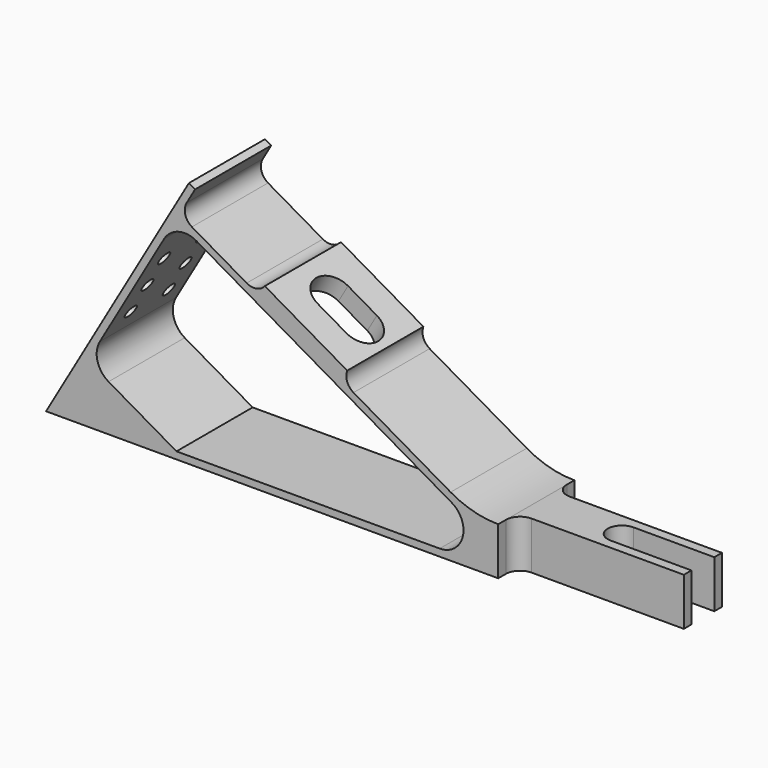
from build123d import *

# Parameters (mm, degrees)
F1_DEPTH    = 10
F2_T1_DEPTH = 20
F4_DEPTH    = 20.001
F5_W        = 35
F5_H        = 5
F6_DEPTH    = 10.001
F7_R        = 3
F9_DEPTH    = 10.001
F11_DEPTH   = 4
F12_R       = 5.5
F13_DEPTH   = 2
F14_R       = 4.25
F15_DEPTH   = 112.584302492
F16_R       = 1.395
F17_DEPTH   = 25


# Not quite as in the source:
# - a fillet or chamfer that OpenCascade refuses, or shapes differently, is made with other operations: its cross-section is extruded or revolved along the edge and cut away or added


with BuildPart() as f1:
    # F0 (on Front) → F1 (new body, symmetric)
    with BuildSketch(Plane.XZ):
        with BuildLine():
            Line((30, 51.9615242271), (0, 0))
            Line((0, 0), (130, 0))
            Line((130, 0), (130, 10))
            Line((130, 10), (95, 10))
            ThreePointArc((95, 10), (89.8236190979, 10.6814834742), (85, 12.6794919243))
            Line((85, 12.6794919243), (62.0314784198, 25.9403740415))
            Line((62.0314784198, 25.9403740415), (63.2814784198, 28.105437551))
            Line((63.2814784198, 28.105437551), (45.9609703441, 38.105437551))
            Line((45.9609703441, 38.105437551), (44.7109703441, 35.9403740415))
            Line((44.7109703441, 35.9403740415), (28.0394191624, 45.5656986041))
            Line((28.0394191624, 45.5656986041), (31.2990381057, 51.2115242271))
            Line((31.2990381057, 51.2115242271), (30, 51.9615242271))
        make_face()
    extrude(amount=F1_DEPTH, both=True)

    # F2: fillet of radius 3 on 3 edges, made by hand

    # F2_s2 → F2_t1 (join)
    with BuildSketch(Plane.XZ.offset(-10)):
        with BuildLine():
            ThreePointArc((63.2814784198, 28.105437551), (63.2705212044, 26.0433626604), (64.5932161113, 24.4613540958))
            Line((64.5932161113, 24.4613540958), (62.0314784198, 25.9403740415))
            Line((62.0314784198, 25.9403740415), (63.2814784198, 28.105437551))
        make_face()
        with BuildLine():
            ThreePointArc((42.1492326526, 37.4193939873), (44.180639712, 37.0649108788), (45.9609703441, 38.105437551))
            Line((45.9609703441, 38.105437551), (44.7109703441, 35.9403740415))
            Line((44.7109703441, 35.9403740415), (42.1492326526, 37.4193939873))
        make_face()
        with BuildLine():
            ThreePointArc((29.5394191624, 48.1637748154), (29.2397178949, 45.8873176801), (30.6374953738, 44.0656986041))
            Line((30.6374953738, 44.0656986041), (28.0394191624, 45.5656986041))
            Line((28.0394191624, 45.5656986041), (29.5394191624, 48.1637748154))
        make_face()
    extrude(amount=F2_T1_DEPTH)

    # F3 (on face) → F4 (cut, through all)
    with BuildSketch(Plane.XZ.offset(10)):
        with BuildLine():
            ThreePointArc((82.7031939779, 1.5), (87.5328231093, 5.2059047745), (85.2031939779, 10.8301270189))
            Line((85.2031939779, 10.8301270189), (31.6195461814, 41.7666604984))
            ThreePointArc((31.6195461814, 41.7666604984), (27.8254509559, 42.2661626109), (24.7894191624, 39.9365334795))
            Line((24.7894191624, 39.9365334795), (11.2990381057, 16.5705080757))
            ThreePointArc((11.2990381057, 16.5705080757), (10.7995359932, 12.7764128502), (13.1291651246, 9.7403810568))
            Line((13.1291651246, 9.7403810568), (27.4019237886, 1.5))
            Line((27.4019237886, 1.5), (82.7031939779, 1.5))
        make_face()
    extrude(amount=-F4_DEPTH, mode=Mode.SUBTRACT)

    # F5 (on face) → F6 (cut, through all)
    with BuildSketch(Plane.XY.offset(10)):
        with Locations((112.5, 7.5)):
            Rectangle(F5_W, F5_H)
        with Locations((112.5, -7.5)):
            Rectangle(F5_W, F5_H)
    extrude(amount=-F6_DEPTH, mode=Mode.SUBTRACT)

    # F7
    f7_edges = [f1.edges().sort_by_distance(p)[0] for p in [
        (95, -5, 5),
        (95, 5, 5),
    ]]
    fillet(f7_edges, radius=F7_R)

    # F8 (on face) → F9 (cut, through all)
    with BuildSketch(Plane.XY.offset(10)):
        with BuildLine():
            Line((130, -3), (130, 3))
            Line((130, 3), (113, 3))
            ThreePointArc((113, 3), (110, 0), (113, -3))
            Line((113, -3), (130, -3))
        make_face()
    extrude(amount=-F9_DEPTH, mode=Mode.SUBTRACT)

    # F10 (on face) → F11 (cut)
    with BuildSketch(Plane(origin=(27.9903810568, 0, 48.4807621135), x_dir=(0.8660254038, 0, -0.5), z_dir=(0.5, 0, 0.8660254038))):
        with BuildLine():
            Line((35, 4), (28, 4))
            ThreePointArc((28, 4), (24, 0), (28, -4))
            Line((28, -4), (35, -4))
            ThreePointArc((35, -4), (39, 0), (35, 4))
        make_face()
    extrude(amount=-F11_DEPTH, mode=Mode.SUBTRACT)

    # F12 (on face) → F13 (cut)
    with BuildSketch(Plane(origin=(0, 0, 0), x_dir=(0, -1, 0), z_dir=(-0.8660254038, 0, 0.5))):
        with Locations((0, 7.5)):
            Circle(F12_R)
    extrude(amount=-F13_DEPTH, mode=Mode.SUBTRACT)

    # F14 (on face) → F15 (cut, through all)
    with BuildSketch(Plane(origin=(0, 0, 0), x_dir=(0, -1, 0), z_dir=(-0.8660254038, 0, 0.5))):
        with Locations((0, 7.5)):
            Circle(F14_R)
    extrude(amount=-F15_DEPTH, mode=Mode.SUBTRACT)

    # F16 (on face) → F17 (cut)
    with BuildSketch(Plane(origin=(0, 0, 0), x_dir=(0, -1, 0), z_dir=(-0.8660254038, 0, 0.5))):
        with Locations((-5, 25)):
            Circle(F16_R)
        with Locations((-5, 32)):
            Circle(F16_R)
        with Locations((-5, 39)):
            Circle(F16_R)
        with Locations((5, 39)):
            Circle(F16_R)
        with Locations((5, 32)):
            Circle(F16_R)
        with Locations((5, 25)):
            Circle(F16_R)
    extrude(amount=-F17_DEPTH, mode=Mode.SUBTRACT)


solid = f1.part
